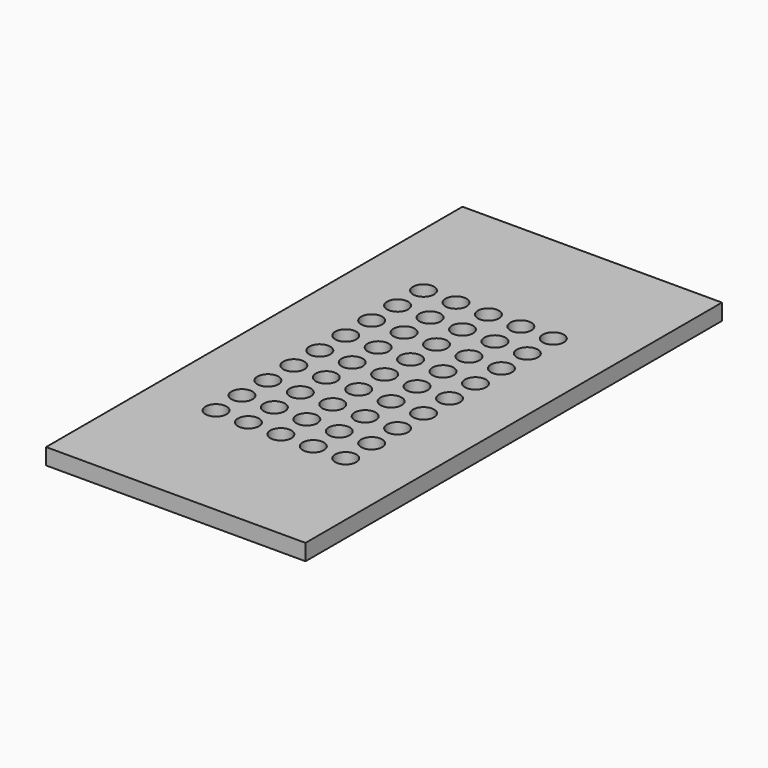
from build123d import *

# Parameters (mm, degrees)
F0_W     = 80
F0_H     = 160.5
F0_R     = 3.25
F1_DEPTH = 5


# Not quite as in the source:
# - a feature of the source that left no trace in its solid (it failed there, or was rolled back) is left out


with BuildPart() as f1:
    # F0 (on Top) → F1 (new body)
    with BuildSketch(Plane.XY):
        Rectangle(F0_W, F0_H)
        with Locations((-20, -39.75)):
            Circle(F0_R, mode=Mode.SUBTRACT)
        with Locations((-20, -29.75)):
            Circle(F0_R, mode=Mode.SUBTRACT)
        with Locations((-10, -39.75)):
            Circle(F0_R, mode=Mode.SUBTRACT)
        with Locations((-10, -29.75)):
            Circle(F0_R, mode=Mode.SUBTRACT)
        with Locations((-20, -19.75)):
            Circle(F0_R, mode=Mode.SUBTRACT)
        with Locations((-20, -9.75)):
            Circle(F0_R, mode=Mode.SUBTRACT)
        with Locations((-10, -19.75)):
            Circle(F0_R, mode=Mode.SUBTRACT)
        with Locations((-10, -9.75)):
            Circle(F0_R, mode=Mode.SUBTRACT)
        with Locations((0, -39.75)):
            Circle(F0_R, mode=Mode.SUBTRACT)
        with Locations((0, -29.75)):
            Circle(F0_R, mode=Mode.SUBTRACT)
        with Locations((10, -39.75)):
            Circle(F0_R, mode=Mode.SUBTRACT)
        with Locations((10, -29.75)):
            Circle(F0_R, mode=Mode.SUBTRACT)
        with Locations((0, -19.75)):
            Circle(F0_R, mode=Mode.SUBTRACT)
        with Locations((0, -9.75)):
            Circle(F0_R, mode=Mode.SUBTRACT)
        with Locations((10, -19.75)):
            Circle(F0_R, mode=Mode.SUBTRACT)
        with Locations((10, -9.75)):
            Circle(F0_R, mode=Mode.SUBTRACT)
        with Locations((20, -39.75)):
            Circle(F0_R, mode=Mode.SUBTRACT)
        with Locations((20, -29.75)):
            Circle(F0_R, mode=Mode.SUBTRACT)
        with Locations((20, -19.75)):
            Circle(F0_R, mode=Mode.SUBTRACT)
        with Locations((20, -9.75)):
            Circle(F0_R, mode=Mode.SUBTRACT)
        with Locations((-20, 0.25)):
            Circle(F0_R, mode=Mode.SUBTRACT)
        with Locations((-20, 10.25)):
            Circle(F0_R, mode=Mode.SUBTRACT)
        with Locations((-10, 0.25)):
            Circle(F0_R, mode=Mode.SUBTRACT)
        with Locations((-10, 10.25)):
            Circle(F0_R, mode=Mode.SUBTRACT)
        with Locations((-20, 20.25)):
            Circle(F0_R, mode=Mode.SUBTRACT)
        with Locations((-20, 30.25)):
            Circle(F0_R, mode=Mode.SUBTRACT)
        with Locations((-10, 20.25)):
            Circle(F0_R, mode=Mode.SUBTRACT)
        with Locations((-10, 30.25)):
            Circle(F0_R, mode=Mode.SUBTRACT)
        with Locations((-20, 40.25)):
            Circle(F0_R, mode=Mode.SUBTRACT)
        with Locations((-10, 40.25)):
            Circle(F0_R, mode=Mode.SUBTRACT)
        with Locations((0, 0.25)):
            Circle(F0_R, mode=Mode.SUBTRACT)
        with Locations((0, 10.25)):
            Circle(F0_R, mode=Mode.SUBTRACT)
        with Locations((10, 0.25)):
            Circle(F0_R, mode=Mode.SUBTRACT)
        with Locations((10, 10.25)):
            Circle(F0_R, mode=Mode.SUBTRACT)
        with Locations((0, 20.25)):
            Circle(F0_R, mode=Mode.SUBTRACT)
        with Locations((0, 30.25)):
            Circle(F0_R, mode=Mode.SUBTRACT)
        with Locations((10, 20.25)):
            Circle(F0_R, mode=Mode.SUBTRACT)
        with Locations((10, 30.25)):
            Circle(F0_R, mode=Mode.SUBTRACT)
        with Locations((20, 0.25)):
            Circle(F0_R, mode=Mode.SUBTRACT)
        with Locations((20, 10.25)):
            Circle(F0_R, mode=Mode.SUBTRACT)
        with Locations((20, 20.25)):
            Circle(F0_R, mode=Mode.SUBTRACT)
        with Locations((20, 30.25)):
            Circle(F0_R, mode=Mode.SUBTRACT)
        with Locations((0, 40.25)):
            Circle(F0_R, mode=Mode.SUBTRACT)
        with Locations((10, 40.25)):
            Circle(F0_R, mode=Mode.SUBTRACT)
        with Locations((20, 40.25)):
            Circle(F0_R, mode=Mode.SUBTRACT)
    extrude(amount=F1_DEPTH)


solid = f1.part
